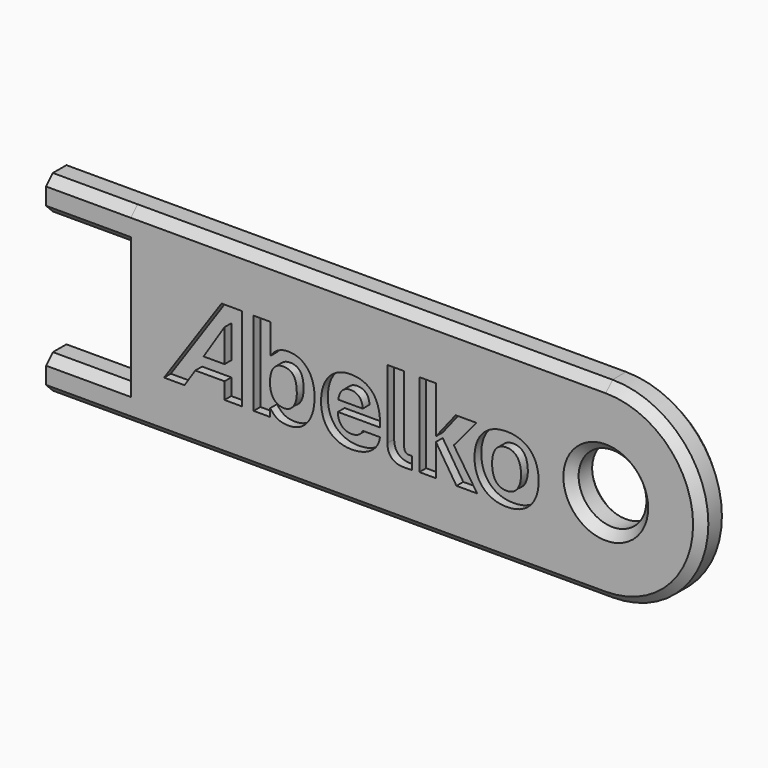
from build123d import *

# Parameters (mm, degrees)
F0_R     = 2
F1_DEPTH = 2
F3_DEPTH = 0.5
F6_DEPTH = 5
F7_SIZE  = 0.49999


# Not quite as in the source:
# - a fillet or chamfer is up to 0.001 mm smaller than in the source, because OpenCascade refuses the exact size
# - a feature names something its author has since deleted; it is built from what else it names


with BuildPart() as f1:
    # F0 (on Front) → F1 (new body)
    with BuildSketch(Plane.XZ):
        with BuildLine():
            Line((-18, 5.15), (-13, 5.15))
            Line((-13, 5.15), (-13, -2.15))
            Line((-13, -2.15), (-18, -2.15))
            Line((-18, -2.15), (-18, -4.15))
            Line((-18, -4.15), (15, -4.15))
            ThreePointArc((15, -4.15), (20.65, 1.5), (15, 7.15))
            Line((15, 7.15), (-18, 7.15))
            Line((-18, 7.15), (-18, 5.15))
        make_face()
        with Locations((15, 1.5)):
            Circle(F0_R, mode=Mode.SUBTRACT)
    extrude(amount=F1_DEPTH)

    # F2 (on face) → F3 (cut)
    with BuildSketch(Plane.XZ.offset(2)):
        Polygon((-6.4611563108, -1.0079550547), (-6.4611104663, 3.943059476), (-7.6544608052, 3.943059476), (-11.0437756499, -1.0079550547), (-9.8374226558, -1.0079550547), (-9.200951568, -0.0383489504), (-7.4783776914, -0.0383489504), (-7.4783776914, -1.0079550547), align=None)
        Polygon((-7.4783776914, 0.8486796922), (-8.7143920972, 0.8486796922), (-7.4783776914, 2.7703563678), align=None, mode=Mode.SUBTRACT)
        with BuildLine():
            add(Edge.make_bspline(
                [(-4.7631894864, 2.1669850315), (-4.5225056976, 2.5245150692), (-4.1993017526, 2.7308727653), (-3.7111148009, 2.7308727653)],
                knots=[0, 0, 0, 0, 1, 1, 1, 1], degree=3))
            Line((-4.7631894864, 2.1669850315), (-4.7631894864, 3.927357724))
            Line((-4.7631894864, 3.927357724), (-5.7603080401, 3.927357724))
            Line((-5.7603080401, 3.927357724), (-5.7603080401, -1.0167973187))
            Line((-5.7603080401, -1.0167973187), (-4.7838195254, -1.0167973187))
            Line((-4.7838195254, -1.0167973187), (-4.7838195254, -0.5561170858))
            add(Edge.make_bspline(
                [(-3.6973614416, -1.1130536425), (-4.1993017526, -1.1130536425), (-4.4812456195, -0.9686490998), (-4.7838195254, -0.5561170858)],
                knots=[0, 0, 0, 0, 1, 1, 1, 1], degree=3))
            add(Edge.make_bspline(
                [(-2.1707958582, 0.8604731979), (-2.1707958582, -0.4666858665), (-2.8515298409, -1.1130536425), (-3.6973614416, -1.1130536425)],
                knots=[0, 0, 0, 0, 1, 1, 1, 1], degree=3))
            add(Edge.make_bspline(
                [(-3.7111148009, 2.7308727653), (-2.8171464425, 2.7308727653), (-2.1707958582, 2.0363281176), (-2.1707958582, 0.8604731979)],
                knots=[0, 0, 0, 0, 1, 1, 1, 1], degree=3))
        make_face()
        with BuildLine():
            add(Edge.make_bspline(
                [(-3.9724286288, -0.2947688745), (-3.5529511683, -0.2947688745), (-3.2159938639, 0.0352945585), (-3.2159938639, 0.7504520535)],
                knots=[0, 0, 0, 0, 1, 1, 1, 1], degree=3))
            add(Edge.make_bspline(
                [(-4.7975728848, 0.7573230027), (-4.7975728848, 0.1109609572), (-4.4881796048, -0.2947688745), (-3.9724286288, -0.2947688745)],
                knots=[0, 0, 0, 0, 1, 1, 1, 1], degree=3))
            add(Edge.make_bspline(
                [(-4.0067547215, 1.8575344459), (-4.5362590569, 1.8575344459), (-4.7975728848, 1.4518218059), (-4.7975728848, 0.7573230027)],
                knots=[0, 0, 0, 0, 1, 1, 1, 1], degree=3))
            add(Edge.make_bspline(
                [(-3.2159938639, 0.7504520535), (-3.2159938639, 1.5275053963), (-3.4910610511, 1.8575344459), (-4.0067547215, 1.8575344459)],
                knots=[0, 0, 0, 0, 1, 1, 1, 1], degree=3))
        make_face(mode=Mode.SUBTRACT)
        with BuildLine():
            add(Edge.make_bspline(
                [(-0.0526639052, 2.744568819), (1.0544242177, 2.744568819), (1.7351582004, 2.0775881956), (1.6938981223, 0.5441058186)],
                knots=[0, 0, 0, 0, 1, 1, 1, 1], degree=3))
            add(Edge.make_bspline(
                [(-1.785529879, 0.7848583742), (-1.785529879, 2.0156980785), (-1.0566591386, 2.744568819), (-0.0526639052, 2.744568819)],
                knots=[0, 0, 0, 0, 1, 1, 1, 1], degree=3))
            add(Edge.make_bspline(
                [(0.0092262119, -1.1405660918), (-0.8434820685, -1.1405660918), (-1.785529879, -0.6386028585), (-1.785529879, 0.7848583742)],
                knots=[0, 0, 0, 0, 1, 1, 1, 1], degree=3))
            add(Edge.make_bspline(
                [(1.6870214426, 0.0421253936), (1.6251313255, -0.5973026665), (1.0337941786, -1.1405660918), (0.0092262119, -1.1405660918)],
                knots=[0, 0, 0, 0, 1, 1, 1, 1], degree=3))
            Line((1.6870214426, 0.0421253936), (0.6624534759, 0.0421253936))
            add(Edge.make_bspline(
                [(0.0160455859, -0.3360690666), (0.2705400398, -0.3360690666), (0.5455499213, -0.2466435779), (0.6624534759, 0.0421253936)],
                knots=[0, 0, 0, 0, 1, 1, 1, 1], degree=3))
            add(Edge.make_bspline(
                [(-0.7953453107, 0.5441058186), (-0.788468631, 0.0352945585), (-0.5202781235, -0.3360690666), (0.0160455859, -0.3360690666)],
                knots=[0, 0, 0, 0, 1, 1, 1, 1], degree=3))
            Line((-0.7953453107, 0.5441058186), (1.6938981223, 0.5441058186))
        make_face()
        with BuildLine():
            add(Edge.make_bspline(
                [(0.6693301556, 1.1905423614), (0.6487001165, 1.6443344535), (0.4011969537, 1.933235228), (-0.0457872255, 1.933235228)],
                knots=[0, 0, 0, 0, 1, 1, 1, 1], degree=3))
            Line((0.6693301556, 1.1905423614), (-0.767838592, 1.1905423614))
            add(Edge.make_bspline(
                [(-0.0457872255, 1.933235228), (-0.4652646861, 1.933235228), (-0.7059484749, 1.6512741694), (-0.767838592, 1.1905423614)],
                knots=[0, 0, 0, 0, 1, 1, 1, 1], degree=3))
        make_face(mode=Mode.SUBTRACT)
        with BuildLine():
            add(Edge.make_bspline(
                [(3.3833837085, -0.3222813238), (3.4383971459, -0.3222813238), (3.5277366761, -0.3222813238), (3.5689967542, -0.3153416079)],
                knots=[0, 0, 0, 0, 1, 1, 1, 1], degree=3))
            add(Edge.make_bspline(
                [(3.1151358953, 0.0215526602), (3.1151358953, -0.2122831017), (3.2183433962, -0.3222813238), (3.3833837085, -0.3222813238)],
                knots=[0, 0, 0, 0, 1, 1, 1, 1], degree=3))
            Line((3.1151358953, 0.0215526602), (3.1151358953, 3.9342344037))
            Line((3.1151358953, 3.9342344037), (2.1249513269, 3.9342344037))
            Line((2.1249513269, 3.9342344037), (2.1249513269, -0.1228518825))
            add(Edge.make_bspline(
                [(3.1151358953, -1.0649283459), (2.3656351158, -1.0649283459), (2.1249513269, -0.6180129335), (2.1249513269, -0.1228518825)],
                knots=[0, 0, 0, 0, 1, 1, 1, 1], degree=3))
            add(Edge.make_bspline(
                [(3.5689967542, -1.0580975107), (3.4177098012, -1.0649283459), (3.2664801539, -1.0649283459), (3.1151358953, -1.0649283459)],
                knots=[0, 0, 0, 0, 1, 1, 1, 1], degree=3))
            Line((3.5689967542, -1.0580975107), (3.5689967542, -0.3153416079))
        make_face()
        Polygon((4.9878276893, 1.1561131185), (4.9878276893, 3.9136043647), (4.0113964803, 3.9136043647), (4.0113964803, -1.0167973187), (4.9878276893, -1.0167973187), (4.9878276893, 0.8673498775), (6.1980660074, -1.0167973187), (7.4220576849, -1.0167973187), (6.0399023747, 1.0392668696), (7.3739782328, 2.6345419441), (6.1499292496, 2.6345419441), align=None)
        with BuildLine():
            add(Edge.make_bspline(
                [(9.1528033491, 2.7652561637), (10.3630416672, 2.7652561637), (11.0437756499, 2.0088213988), (11.0437756499, 0.7985830807)],
                knots=[0, 0, 0, 0, 1, 1, 1, 1], degree=3))
            add(Edge.make_bspline(
                [(7.2617737426, 0.8122791344), (7.2617737426, 1.940054602), (7.928754366, 2.7652561637), (9.1528033491, 2.7652561637)],
                knots=[0, 0, 0, 0, 1, 1, 1, 1], degree=3))
            add(Edge.make_bspline(
                [(9.1596800288, -1.1474141187), (7.9700144441, -1.1474141187), (7.2617737426, -0.3497708508), (7.2617737426, 0.8122791344)],
                knots=[0, 0, 0, 0, 1, 1, 1, 1], degree=3))
            add(Edge.make_bspline(
                [(11.0437756499, 0.7985830807), (11.0437756499, -0.3222813238), (10.4042444396, -1.1474141187), (9.1596800288, -1.1474141187)],
                knots=[0, 0, 0, 0, 1, 1, 1, 1], degree=3))
        make_face()
        with BuildLine():
            add(Edge.make_bspline(
                [(9.1528033491, -0.3153416079), (9.6753736992, -0.3153416079), (10.0053970182, 0.090319457), (10.0053970182, 0.7985830807)],
                knots=[0, 0, 0, 0, 1, 1, 1, 1], degree=3))
            add(Edge.make_bspline(
                [(8.3000950687, 0.8122791344), (8.3000950687, 0.0628528523), (8.6163650284, -0.3153416079), (9.1528033491, -0.3153416079)],
                knots=[0, 0, 0, 0, 1, 1, 1, 1], degree=3))
            add(Edge.make_bspline(
                [(9.1528033491, 1.933235228), (8.7539559276, 1.933235228), (8.3000950687, 1.7337599422), (8.3000950687, 0.8122791344)],
                knots=[0, 0, 0, 0, 1, 1, 1, 1], degree=3))
            add(Edge.make_bspline(
                [(10.0053970182, 0.7985830807), (10.0053970182, 1.5618429502), (9.6615630342, 1.933235228), (9.1528033491, 1.933235228)],
                knots=[0, 0, 0, 0, 1, 1, 1, 1], degree=3))
        make_face(mode=Mode.SUBTRACT)
    extrude(amount=-F3_DEPTH, mode=Mode.SUBTRACT)

    # F4 (on face) + F5 (on face) → F6 (cut)
    with BuildSketch(Plane(origin=(-18, 0, 0), x_dir=(0, -1, 0), z_dir=(-1, 0, 0))):
        Polygon((0.5, 5.15), (0, 5.65), (0, 5.15), align=None)
        Polygon((0, 7.15), (0, 6.65), (0.5, 7.15), align=None)
        Polygon((2, 7.15), (1.5, 7.15), (2, 6.65), align=None)
        Polygon((2, 5.65), (1.5, 5.15), (2, 5.15), align=None)
    with BuildSketch(Plane(origin=(-18, 0, 0), x_dir=(0, -1, 0), z_dir=(-1, 0, 0))):
        Polygon((0, -2.15), (0, -2.65), (0.5, -2.15), align=None)
        Polygon((2, -2.15), (1.5, -2.15), (2, -2.65), align=None)
        Polygon((2, -3.65), (1.5, -4.15), (2, -4.15), align=None)
        Polygon((0.5, -4.15), (0, -3.65), (0, -4.15), align=None)
    extrude(amount=-F6_DEPTH, mode=Mode.SUBTRACT)

    # F7 (size 0.5 in the source; OpenCascade refuses exactly that, so slightly less here)
    f7_edges = [f1.edges().sort_by_distance(p)[0] for p in [
        (1, -2, -4.15),
        (20.65, -2, 1.5),
        (1, -2, 7.15),
        (1, 0, -4.15),
        (13, -2, 1.5),
        (13, 0, 1.5),
    ]]
    chamfer(f7_edges, length=F7_SIZE)


solid = f1.part
